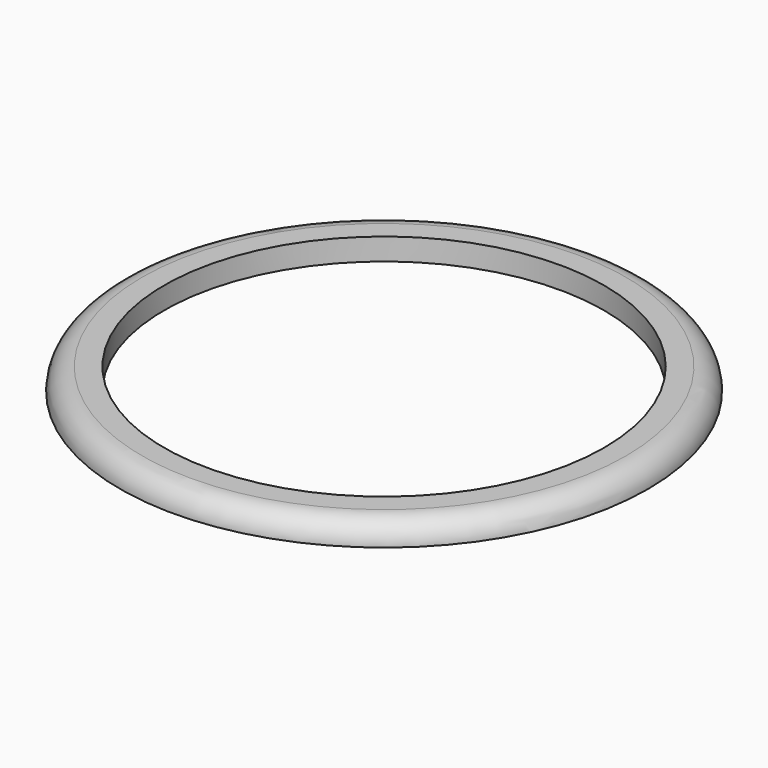
from build123d import *

# Parameters (mm, degrees)
F0_R     = 60.96
F0_R_2   = 50.8
F1_DEPTH = 5.08
F2_R     = 5.07999


# Not quite as in the source:
# - a fillet or chamfer is up to 0.001 mm smaller than in the source, because OpenCascade refuses the exact size


with BuildPart() as f1:
    # F0 (on Top) → F1 (new body)
    with BuildSketch(Plane.XY):
        Circle(F0_R)
        Circle(F0_R_2, mode=Mode.SUBTRACT)
    extrude(amount=F1_DEPTH)

    # F2 (radius 5.08 in the source; OpenCascade refuses exactly that, so slightly less here)
    f2_edges = [f1.edges().sort_by_distance(p)[0] for p in [
        (-60.96, 0, 5.08),
    ]]
    fillet(f2_edges, radius=F2_R)


solid = f1.part
